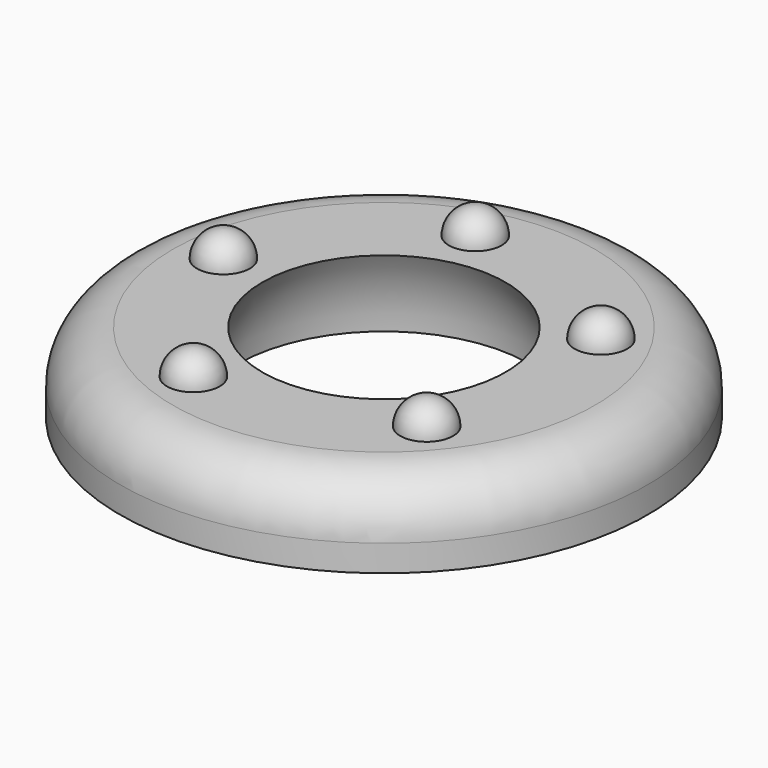
from build123d import *

# Parameters (mm, degrees)
F2_R     = 2
F3_R     = 1
F4_DEPTH = 1
F5_R     = 0.99999
F6_COUNT = 5


# Not quite as in the source:
# - a fillet or chamfer is up to 0.001 mm smaller than in the source, because OpenCascade refuses the exact size


with BuildPart() as f1:
    # F0 (on Front) → F1 (revolve)
    with BuildSketch(Plane.XZ):
        with BuildLine():
            ThreePointArc((-5.5, 0), (-5.2727482046, 1.564648961), (-4.6097722286, 3))
            Line((-4.6097722286, 3), (-10, 3))
            Line((-10, 3), (-10, 0))
            Line((-10, 0), (-5.5, 0))
        make_face()
    revolve(axis=Axis((0, 0, 1.7619796563), (0, 0, 1)))

    # F2
    f2_edges = [f1.edges().sort_by_distance(p)[0] for p in [
        (10, 0, 3),
    ]]
    fillet(f2_edges, radius=F2_R)

    # F3 (on face) → F4 (join)
    with BuildSketch(Plane.XY.offset(3)):
        with Locations((-6.4481133595, 0.457114249)):
            Circle(F3_R)
    extrude(amount=F4_DEPTH)

    # F5 (radius 1 in the source; OpenCascade refuses exactly that, so slightly less here)
    f5_edges = [f1.edges().sort_by_distance(p)[0] for p in [
        (-7.448113, 0.457114, 4),
    ]]
    fillet(f5_edges, radius=F5_R)

    # F6: F1 ×5 about axis
    f6_axis = Axis((0, 0, 3), (0, 0, 1))


with BuildPart() as f1_1:
    add(f1.part)
    for i in range(1, F6_COUNT):
        add(f1.part.rotate(f6_axis, i * 360 / F6_COUNT))


solid = f1_1.part
